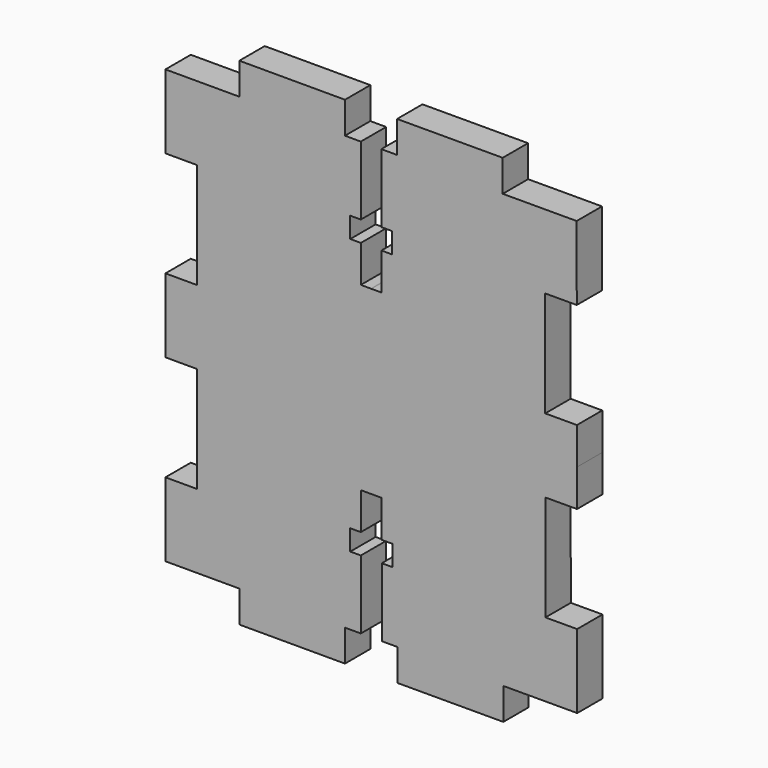
from build123d import *

# Parameters (mm, degrees)
F1_DEPTH = 3


# Not quite as in the source:
# - ends of sketch curves that miss each other by under 0.0002 mm in the source are joined


with BuildPart() as f1:
    # F0 (on Front) → F1 (new body)
    with BuildSketch(Plane.XZ):
        Polygon((3, 24), (0, 24), (0, 20.5), (0, 17), (3, 17), (2.9999999981, 7), (0, 7), (-2.3e-09, 0), (7, 0), (6.9999999985, -3), (17, -3), (16.9999999997, 0), (18.5, 0), (18.4999999999, 6.5), (17.5, 6.5), (17.5, 8.446655035), (18.5, 8.446655035), (18.4999999999, 11.946655035), (19.4755076583, 11.946655035), (19.5, 11.946655035), (20.4755068041, 11.9479460792), (20.4800814811, 8.4479490688), (21.480081481, 8.4479490688), (21.4826258575, 6.5012956966), (20.4826258575, 6.5012956966), (20.4911216861, 0.0013012489), (21.9911204047, 0.0032618247), (21.9950415565, -2.9967356127), (31.9950330143, -2.9836651074), (31.9911118642, 0.01633233), (38.9911058834, 0.0254816838), (38.981956532, 7.0254757044), (35.9819590922, 7.0215545528), (35.9688885888, 17.0215460109), (38.9688860243, 17.0254671625), (38.9643113475, 20.5254641728), (38.9597366706, 24.0254611832), (35.9597392332, 24.0215400316), (35.9466687298, 34.0215314897), (38.9466661653, 34.0254526413), (38.9375168138, 41.0254466619), (31.9375227909, 41.0162973082), (31.9336016407, 44.0162947456), (21.9336101812, 44.0032242403), (21.9375313331, 41.0032268029), (20.4375326141, 41.0012662271), (20.4460284426, 34.5012717793), (21.4460275885, 34.5025788298), (21.4460275882, 32.555922132), (20.448572819, 32.5546184071), (20.453147496, 29.0546213968), (19.49999996, 29.0533755837), (19.4531483501, 29.053344965), (18.5, 29.053344965), (18.5, 32.553344965), (17.5, 32.553344965), (17.5, 34.5), (18.5, 34.5), (18.5, 41), (17, 41), (17, 44), (7, 44), (7, 41), (0, 41), (0, 34), (3, 34), align=None)
    extrude(amount=F1_DEPTH)


solid = f1.part
